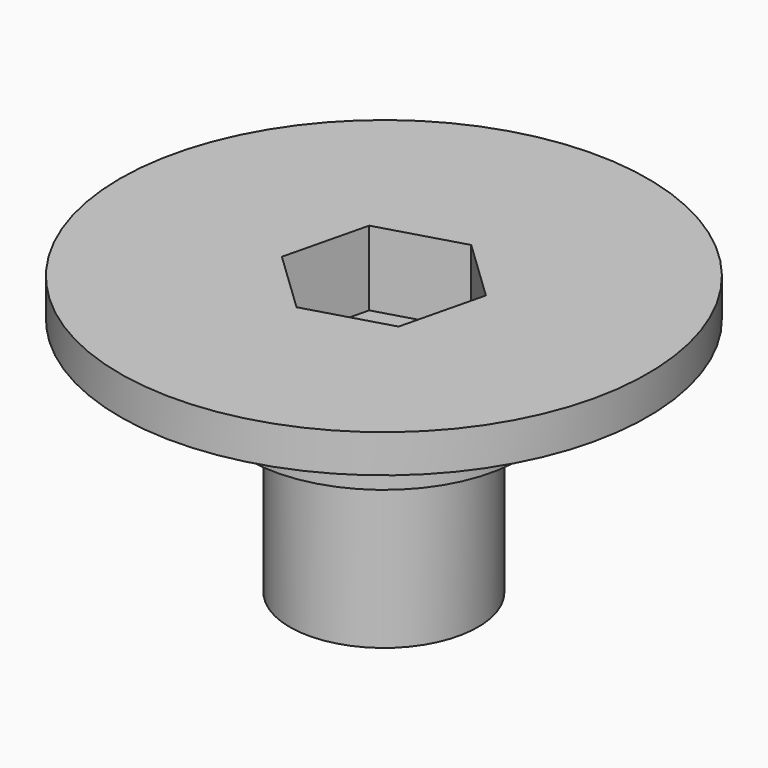
from build123d import *

# Parameters (mm, degrees)
F0_W     = 0.7
F0_H     = 7.9574310766
F2_R     = 3.525
F3_DEPTH = 6.5


# Not quite as in the source:
# - a feature names something its author has since deleted; it is built from what else it names


with BuildPart() as f1:
    # F0 (on Front) → F1 (revolve)
    with BuildSketch(Plane.XZ):
        Polygon((-8.2, 24.3467036635), (-8.2, 18.3), (-7.5, 18.3), (-7.5, 20.7), (-7.5, 27), (-3.525, 27), (-3.525, 28.3), (-3.525, 34.6), (-23, 34.6), (-23, 31.2892384827), (-11.8090426549, 31.2892384827), (-11.8090426549, 26.945874095), (-11.8090426549, 24.3467036635), align=None)
        with Locations((-7.85, 14.3212844617)):
            Rectangle(F0_W, F0_H)
    revolve(axis=Axis((0, 0, 19.15), (0, 0, -1)))

    # F2 (on face) → F3 (cut)
    with BuildSketch(Plane.XY.offset(34.6)):
        Polygon((-7.2035379805, -2.107693976), (-1.7764524637, -7.2922938762), (5.4270855169, -5.1845999003), (7.2035379805, 2.107693976), (1.7764524637, 7.2922938762), (-5.4270855169, 5.1845999003), align=None)
        Circle(F2_R, mode=Mode.SUBTRACT)
    extrude(amount=-F3_DEPTH, mode=Mode.SUBTRACT)


solid = f1.part
